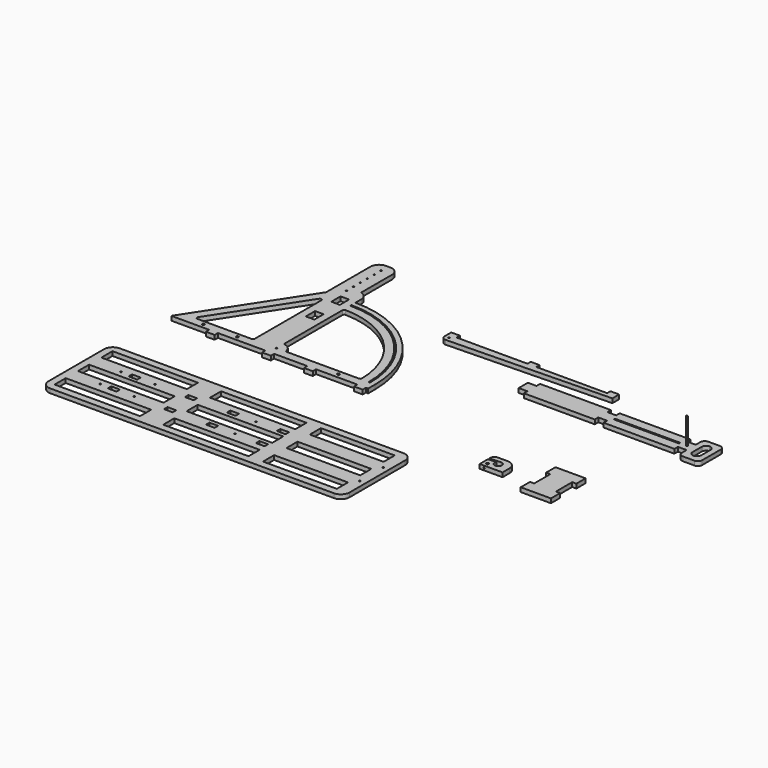
from build123d import *

# Parameters (mm, degrees)
F0_R          = 5.334
F0_W          = 37.592
F0_H          = 50.8
F0_R_2        = 3.302
F0_W_2        = 38.1
F0_H_2        = 18.034
F1_DEPTH      = 18.796
F0_R_3        = 3.3655
F0_W_3        = 285.75
F0_H_3        = 6.604
F0_H_4        = 88.9
F0_W_4        = 374.9063185829
F0_H_5        = 61.0004067421
F0_H_6        = 19.304
F0_W_5        = 375.6683185829
F0_W_6        = 374.3936814171
F0_W_7        = 323.85
F0_R_4        = 3.175
F0_W_8        = 18.288
F2_T1_DEPTH   = 207.0075525849
F2_T3_DEPTH   = 211.6122724423
F2_T5_DEPTH   = 206.6295731852
F2_2_F1_R     = 38.1
F2_2_F2_R     = 38.1
F2_2_F3_R     = 38.1
F2_2_F4_R     = 38.1
F2_3_T1_DEPTH = 209.296
F3_R          = 7.62
F4_R          = 19.04999
F4_2_R        = 19.04999
F5_DEPTH      = 133.858
F6_R          = 3.175
F7_DEPTH      = 22.225


# Not quite as in the source:
# - a fillet or chamfer that OpenCascade refuses, or shapes differently, is made with other operations: its cross-section is extruded or revolved along the edge and cut away or added
# - a fillet or chamfer is up to 0.001 mm smaller than in the source, because OpenCascade refuses the exact size


with BuildPart() as f1:
    # F0 (on Top) → F1 (new body)
    with BuildSketch(Plane.XY):
        with BuildLine():
            Line((-126.9907256682, 429.9398570147), (-431.8, -38.1))
            Line((-431.8, -38.1), (-265.5232921987, -38.1))
            Line((-265.5232921987, -38.1), (-227.4232921987, -38.1))
            Line((-227.4232921987, -38.1), (-19.05, -38.1))
            Line((-19.05, -38.1), (0, -38.1))
            Line((0, -38.1), (19.05, -38.1))
            Line((19.05, -38.1), (165.1, -38.1))
            Line((165.1, -38.1), (203.2, -38.1))
            Line((203.2, -38.1), (384.1496, -38.1))
            Line((384.1496, -38.1), (422.2496, -38.1))
            Line((422.2496, -38.1), (431.8, -38.1))
            Line((431.8, -38.1), (431.8, 0))
            ThreePointArc((431.8, 0), (305.3287081164, 305.3287081164), (0, 431.8))
            Line((0, 431.8), (0, 501.4883419246))
            Line((0, 501.4883419246), (-31.7476814171, 501.4883419246))
            Line((-31.7476814171, 501.4883419246), (-31.7476814171, 571.1766838493))
            Line((-31.7476814171, 571.1766838493), (-31.7476814171, 710.1696690659))
            Line((-31.7476814171, 710.1696690659), (-79.3692035427, 710.7452170149))
            Line((-79.3692035427, 710.7452170149), (-126.9907256682, 711.3207649639))
            Line((-126.9907256682, 711.3207649639), (-126.9907256682, 429.9398570147))
        make_face()
        with Locations((-306.2257121472, -19.05)):
            Circle(F0_R, mode=Mode.SUBTRACT)
        with Locations((-157.5365847975, -19.05)):
            Circle(F0_R, mode=Mode.SUBTRACT)
        with Locations((285.75, -19.05)):
            Circle(F0_R, mode=Mode.SUBTRACT)
        Polygon((-102.2420211227, 398.1261971854), (-102.2420211227, 0), (-361.5202758221, 0), align=None, mode=Mode.SUBTRACT)
        with Locations((-50.5436814171, 271.7317342758)):
            Rectangle(F0_W, F0_H, mode=Mode.SUBTRACT)
        with BuildLine():
            ThreePointArc((3.302, 0), (2.3348665915, -2.3348665915), (0, -3.302))
            ThreePointArc((0, -3.302), (-3.302, 0), (0, 3.302))
            Line((0, 3.302), (0, 38.1))
            Line((0, 38.1), (0, 368.3))
            ThreePointArc((0, 368.3), (260.427427511, 260.427427511), (368.3, 0))
            Line((368.3, 0), (38.1, 0))
            Line((38.1, 0), (3.302, 0))
        make_face(mode=Mode.SUBTRACT)
        with BuildLine():
            ThreePointArc((0, 409.6004), (289.6312204167, 289.6312204167), (409.6004, 0))
            Line((409.6004, 0), (403.1996, 0))
            ThreePointArc((403.1996, 0), (285.1051713317, 285.1051713317), (0, 403.1996))
            Line((0, 403.1996), (0, 409.6004))
        make_face(mode=Mode.SUBTRACT)
        with Locations((-50.5436814171, 411.4317342758)):
            Rectangle(F0_W, F0_H, mode=Mode.SUBTRACT)
        with Locations((-79.8296419019, 482.1479993145)):
            Circle(F0_R_2, mode=Mode.SUBTRACT)
        with Locations((-79.8296419019, 520.2479993145)):
            Circle(F0_R_2, mode=Mode.SUBTRACT)
        with Locations((-79.8296419019, 558.3479993145)):
            Circle(F0_R_2, mode=Mode.SUBTRACT)
        with Locations((-79.8296419019, 596.4479993145)):
            Circle(F0_R_2, mode=Mode.SUBTRACT)
        with BuildLine():
            ThreePointArc((-76.5276419019, 634.5479993145), (-82.1645084933, 632.213132723), (-79.8296419019, 637.8499993145))
            ThreePointArc((-79.8296419019, 637.8499993145), (-77.4947753104, 636.8828659059), (-76.5276419019, 634.5479993145))
        make_face(mode=Mode.SUBTRACT)
        with BuildLine():
            ThreePointArc((-79.8296419019, 669.3459993145), (-83.1315816182, 672.6679520076), (-79.7897372441, 675.9497581818))
            ThreePointArc((-79.7897372441, 675.9497581818), (-77.4807092528, 674.9687145943), (-76.5276419019, 672.6479993145))
            ThreePointArc((-76.5276419019, 672.6479993145), (-77.4947753104, 670.313132723), (-79.8296419019, 669.3459993145))
        make_face(mode=Mode.SUBTRACT)
        with Locations((-246.4732921987, -47.117)):
            Rectangle(F0_W_2, F0_H_2)
        Polygon((0, -38.1), (-19.05, -38.1), (-19.05, -56.134), (19.05, -56.134), (19.05, -38.1), align=None)
        with Locations((403.1996, -47.117)):
            Rectangle(F0_W_2, F0_H_2)
        with Locations((184.15, -47.117)):
            Rectangle(F0_W_2, F0_H_2)
        with BuildLine():
            Line((0, 38.1), (0, 3.302))
            ThreePointArc((0, 3.302), (2.3348665915, 2.3348665915), (3.302, 0))
            Line((3.302, 0), (38.1, 0))
            ThreePointArc((38.1, 0), (26.9407683632, 26.9407683632), (0, 38.1))
        make_face()
    extrude(amount=F1_DEPTH)

    # F2: fillet of radius 38.1 on 3 edges, made by hand

    # F2_s2 → F2_t1 (cut)
    with BuildSketch(Plane.XY.offset(-94.1057762924)):
        with BuildLine():
            ThreePointArc((-31.7476814171, 672.5273585489), (-42.7446123889, 699.3048425468), (-69.3872430578, 710.6245762494))
            Line((-69.3872430578, 710.6245762494), (-31.7476814171, 710.1696690659))
            Line((-31.7476814171, 710.1696690659), (-31.7476814171, 672.5273585489))
        make_face()
    extrude(amount=F2_T1_DEPTH, mode=Mode.SUBTRACT)

    # F2_s4 → F2_t3 (cut)
    with BuildSketch(Plane.XY.offset(-96.4081362212)):
        with BuildLine():
            ThreePointArc((-88.430287309, 710.854728176), (-115.6682096661, 699.8605795036), (-126.9907256682, 672.7575104755))
            Line((-126.9907256682, 672.7575104755), (-126.9907256682, 711.3207649639))
            Line((-126.9907256682, 711.3207649639), (-88.430287309, 710.854728176))
        make_face()
    extrude(amount=F2_T3_DEPTH, mode=Mode.SUBTRACT)

    # F2_s6 → F2_t5 (cut)
    with BuildSketch(Plane.XY.offset(-93.9167865926)):
        with BuildLine():
            ThreePointArc((0, 463.9216272876), (-8.9998854125, 488.5141735363), (-31.7476814171, 501.4883419246))
            Line((-31.7476814171, 501.4883419246), (0, 501.4883419246))
            Line((0, 501.4883419246), (0, 463.9216272876))
        make_face()
    extrude(amount=F2_T5_DEPTH, mode=Mode.SUBTRACT)

    # F3
    f3_edges = [f1.edges().sort_by_distance(p)[0] for p in [
        (-102.242021, 398.126197, 9.398),
        (0, 368.3, 9.398),
        (-361.520276, 0, 9.398),
        (-102.242021, 0, 9.398),
        (0, 38.1, 9.398),
        (38.1, 0, 9.398),
        (368.3, 0, 9.398),
        (-31.747681, 501.488342, 9.398),
    ]]
    fillet(f3_edges, radius=F3_R)


with BuildPart() as f1b:
    # F0 (on Top) → F1, piece 2 (new body)
    with BuildSketch(Plane.XY):
        with BuildLine():
            Line((413.4104257778, 409.7277641083), (1130.5077061616, 427.6877343655))
            Line((1130.5077061616, 427.6877343655), (1130.5077061616, 446.7377343655))
            Line((1130.5077061616, 446.7377343655), (1092.4077061616, 446.7377343655))
            Line((1092.4077061616, 446.7377343655), (781.2577061616, 446.7377343655))
            Line((781.2577061616, 446.7377343655), (743.1577061616, 446.7377343655))
            Line((743.1577061616, 446.7377343655), (432.0077061616, 446.7377343655))
            Line((432.0077061616, 446.7377343655), (393.9077061616, 446.7377343655))
            Line((393.9077061616, 446.7377343655), (393.9077061616, 427.6877343655))
            ThreePointArc((393.9077061616, 427.6877343655), (400.0239381517, 414.7603663856), (413.4104257778, 409.7277641083))
        make_face()
        with Locations((412.9332898804, 428.7786227405)):
            Circle(F0_R_3, mode=Mode.SUBTRACT)
        with Locations((762.2077061616, 455.7547343655)):
            Rectangle(F0_W_2, F0_H_2)
        with Locations((1111.4577061616, 455.7547343655)):
            Rectangle(F0_W_2, F0_H_2)
        with Locations((412.9577061616, 455.7547343655)):
            Rectangle(F0_W_2, F0_H_2)
    extrude(amount=F1_DEPTH)


with BuildPart() as f1c:
    # F0 (on Top) → F1, piece 3 (new body)
    with BuildSketch(Plane.XY):
        Polygon((1181.3658170382, 356.6390027832), (870.2158170382, 356.6390027832), (870.2158170382, 337.3350027832), (832.1158170382, 337.3350027832), (832.1158170382, 287.0430027832), (870.2158170382, 287.0430027832), (870.2158170382, 267.7390027832), (1181.3658170382, 267.7390027832), (1181.3658170382, 287.0430027832), (1219.4658170382, 287.0430027832), (1219.4658170382, 267.7390027832), (1530.6158170382, 267.7390027832), (1530.6158170382, 287.0430027832), (1568.7158170382, 287.0430027832), (1568.7158170382, 267.7390027832), (1568.7158170382, 242.3390027832), (1657.6158170382, 242.3390027832), (1657.6158170382, 382.0390027832), (1568.7158170382, 382.0390027832), (1568.7158170382, 356.6390027832), (1568.7158170382, 337.3350027832), (1530.6158170382, 337.3350027832), (1530.6158170382, 356.6390027832), (1219.4658170382, 356.6390027832), (1219.4658170382, 337.3350027832), (1181.3658170382, 337.3350027832), align=None)
        with Locations((1375.0408170382, 312.1890027832)):
            Rectangle(F0_W_3, F0_H_3, mode=Mode.SUBTRACT)
        with Locations((1549.6658170382, 312.1890027832)):
            Circle(F0_R_2, mode=Mode.SUBTRACT)
        with Locations((1613.1658170382, 313.4407141018)):
            Rectangle(F0_W_2, F0_H_4, mode=Mode.SUBTRACT)
    extrude(amount=F1_DEPTH)

    # F4 (radius 19.05 in the source; OpenCascade refuses exactly that, so slightly less here)
    f4_edges = [f1c.edges().sort_by_distance(p)[0] for p in [
        (1594.115817, 268.990714, 9.398),
        (1657.615817, 242.339003, 9.398),
        (1657.615817, 382.039003, 9.398),
        (1568.715817, 382.039003, 9.398),
        (1568.715817, 242.339003, 9.398),
        (1594.115817, 357.890714, 9.398),
        (1632.215817, 357.890714, 9.398),
        (1632.215817, 268.990714, 9.398),
    ]]
    fillet(f4_edges, radius=F4_R)


with BuildPart() as f1d:
    # F0 (on Top) → F1, piece 4 (new body)
    with BuildSketch(Plane.XY):
        Polygon((457.2, -336.8782309055), (-457.2, -336.8782309055), (-457.2, -479.7532309055), (-457.2, -575.0032309055), (-457.2, -717.8782309055), (457.2, -717.8782309055), (457.2, -575.0032309055), (457.2, -479.7532309055), align=None)
        with Locations((-237.9968407085, -655.6280275345)):
            Rectangle(F0_W_4, F0_H_5, mode=Mode.SUBTRACT)
        with Locations((-306.2257121472, -584.6552309055)):
            Circle(F0_R_2, mode=Mode.SUBTRACT)
        with Locations((-246.4732921987, -584.6552309055)):
            Rectangle(F0_W_2, F0_H_6, mode=Mode.SUBTRACT)
        with Locations((-157.5365847975, -584.6552309055)):
            Circle(F0_R_2, mode=Mode.SUBTRACT)
        with Locations((0, -584.6552309055)):
            Rectangle(F0_W_2, F0_H_6, mode=Mode.SUBTRACT)
        with Locations((-237.6158407085, -527.3782309055)):
            Rectangle(F0_W_5, F0_H_5, mode=Mode.SUBTRACT)
        with Locations((-306.2294371336, -470.1227213125)):
            Circle(F0_R_2, mode=Mode.SUBTRACT)
        with Locations((-246.4732921987, -471.0306376476)):
            Rectangle(F0_W_2, F0_H_6, mode=Mode.SUBTRACT)
        with Locations((-237.9968407085, -399.1284342766)):
            Rectangle(F0_W_4, F0_H_5, mode=Mode.SUBTRACT)
        with Locations((-157.5365847975, -470.1012309055)):
            Circle(F0_R_2, mode=Mode.SUBTRACT)
        with Locations((0, -470.1012309055)):
            Rectangle(F0_W_2, F0_H_6, mode=Mode.SUBTRACT)
        with Locations((238.2531592915, -655.6280275345)):
            Rectangle(F0_W_6, F0_H_5, mode=Mode.SUBTRACT)
        with Locations((184.15, -584.6552309055)):
            Rectangle(F0_W_2, F0_H_6, mode=Mode.SUBTRACT)
        with Locations((285.75, -584.6552309055)):
            Circle(F0_R_2, mode=Mode.SUBTRACT)
        with Locations((403.1996, -584.6552309055)):
            Rectangle(F0_W_2, F0_H_6, mode=Mode.SUBTRACT)
        with Locations((184.15, -470.1012309055)):
            Rectangle(F0_W_2, F0_H_6, mode=Mode.SUBTRACT)
        with Locations((238.8904778744, -527.3782309055)):
            Rectangle(F0_W_5, F0_H_5, mode=Mode.SUBTRACT)
        with Locations((285.75, -470.1012309055)):
            Circle(F0_R_2, mode=Mode.SUBTRACT)
        with Locations((238.2531592915, -399.1284342766)):
            Rectangle(F0_W_6, F0_H_5, mode=Mode.SUBTRACT)
        with Locations((403.1996, -470.1012309055)):
            Rectangle(F0_W_2, F0_H_6, mode=Mode.SUBTRACT)
        Polygon((863.6, -336.8782309055), (457.2, -336.8782309055), (457.2, -479.7532309055), (457.2, -575.0032309055), (457.2, -717.8782309055), (863.6, -717.8782309055), align=None)
        with Locations((650.875, -655.6280275345)):
            Rectangle(F0_W_7, F0_H_5, mode=Mode.SUBTRACT)
        with Locations((838.2, -591.50312922)):
            Circle(F0_R_4, mode=Mode.SUBTRACT)
        with Locations((650.875, -527.3782309055)):
            Rectangle(F0_W_7, F0_H_5, mode=Mode.SUBTRACT)
        with Locations((838.2, -463.2533325911)):
            Circle(F0_R_4, mode=Mode.SUBTRACT)
        with Locations((650.875, -399.1284342766)):
            Rectangle(F0_W_7, F0_H_5, mode=Mode.SUBTRACT)
    extrude(amount=F1_DEPTH)

    # F2#2: fillet of radius 38.1 on 4 edges, made by hand

    # F2_2_f1
    f2_2_f1_edges = [f1d.edges().sort_by_distance(p)[0] for p in [
        (-457.2, -336.8782309055, 9.398),
    ]]
    fillet(f2_2_f1_edges, radius=F2_2_F1_R)

    # F2_2_f2
    f2_2_f2_edges = [f1d.edges().sort_by_distance(p)[0] for p in [
        (-457.2, -717.8782309055, 9.398),
    ]]
    fillet(f2_2_f2_edges, radius=F2_2_F2_R)

    # F2_2_f3
    f2_2_f3_edges = [f1d.edges().sort_by_distance(p)[0] for p in [
        (863.6, -717.8782309055, 9.398),
    ]]
    fillet(f2_2_f3_edges, radius=F2_2_F3_R)

    # F2_2_f4
    f2_2_f4_edges = [f1d.edges().sort_by_distance(p)[0] for p in [
        (863.6, -336.8782309055, 9.398),
    ]]
    fillet(f2_2_f4_edges, radius=F2_2_F4_R)


with BuildPart() as f1e:
    # F0 (on Top) → F1, piece 5 (new body)
    with BuildSketch(Plane.XY):
        with BuildLine():
            Line((1179.8847913742, -160.0811118364), (1079.6542167664, -160.0811118364))
            Line((1079.6542167664, -160.0811118364), (1079.6542167664, -183.9004432114))
            Line((1079.6542167664, -183.9004432114), (1128.7826850275, -180.8406102839))
            ThreePointArc((1128.7826850275, -180.8406102839), (1138.4168071881, -209.9980522555), (1115.695113924, -189.3413974599))
            Line((1115.695113924, -189.3413974599), (1079.6542167664, -191.586106643))
            Line((1079.6542167664, -191.586106643), (1079.6542167664, -236.2811118364))
            Line((1079.6542167664, -236.2811118364), (1179.8847913742, -236.2811118364))
            Line((1179.8847913742, -236.2811118364), (1179.8847913742, -160.0811118364))
        make_face()
        with Locations((1098.7042167664, -217.2311118364)):
            Circle(F0_R, mode=Mode.SUBTRACT)
    extrude(amount=F1_DEPTH)

    # F2#3: fillet of radius 38.1 on 1 edges, made by hand

    # F2_3_s2 → F2_3_t1 (cut)
    with BuildSketch(Plane.XY.offset(-95.25)):
        with BuildLine():
            ThreePointArc((1141.7847913742, -160.0811118364), (1168.7255597374, -171.2403434732), (1179.8847913742, -198.1811118364))
            Line((1179.8847913742, -198.1811118364), (1179.8847913742, -160.0811118364))
            Line((1179.8847913742, -160.0811118364), (1141.7847913742, -160.0811118364))
        make_face()
    extrude(amount=F2_3_T1_DEPTH, mode=Mode.SUBTRACT)

    # F4#2 (radius 19.05 in the source; OpenCascade refuses exactly that, so slightly less here)
    f4_2_edges = [f1e.edges().sort_by_distance(p)[0] for p in [
        (1079.654217, -160.081112, 9.398),
    ]]
    fillet(f4_2_edges, radius=F4_2_R)

    # F6 (on face) → F7 (cut)
    with BuildSketch(Plane.XZ.offset(236.2811118364)):
        with Locations((1098.7042167664, 9.398)):
            Circle(F6_R)
    extrude(amount=-F7_DEPTH, mode=Mode.SUBTRACT)


with BuildPart() as f1f:
    # F0 (on Top) → F1, piece 6 (new body)
    with BuildSketch(Plane.XY):
        Polygon((1411.5280814667, -92.9154240131), (1315.7700814667, -92.9154240131), (1315.7700814667, -143.7154240131), (1315.7700814667, -232.6154240131), (1315.7700814667, -283.4154240131), (1411.5280814667, -283.4154240131), (1411.5280814667, -232.6154240131), (1411.5280814667, -143.7154240131), align=None)
        with Locations((1306.6260814667, -118.3154240131)):
            Rectangle(F0_W_8, F0_H)
        with Locations((1420.6720814667, -118.3154240131)):
            Rectangle(F0_W_8, F0_H)
        with Locations((1306.6260814667, -258.0154240131)):
            Rectangle(F0_W_8, F0_H)
        with Locations((1420.6720814667, -258.0154240131)):
            Rectangle(F0_W_8, F0_H)
    extrude(amount=F1_DEPTH)


with BuildPart() as f5:
    # F0 (on Top) → F5 (new body)
    with BuildSketch(Plane.XY):
        with Locations((1549.6658170382, 312.1890027832)):
            Circle(F0_R_2)
    extrude(amount=F5_DEPTH)


solid = Compound([f1.part, f1b.part, f1c.part, f1d.part, f1e.part, f1f.part, f5.part])
